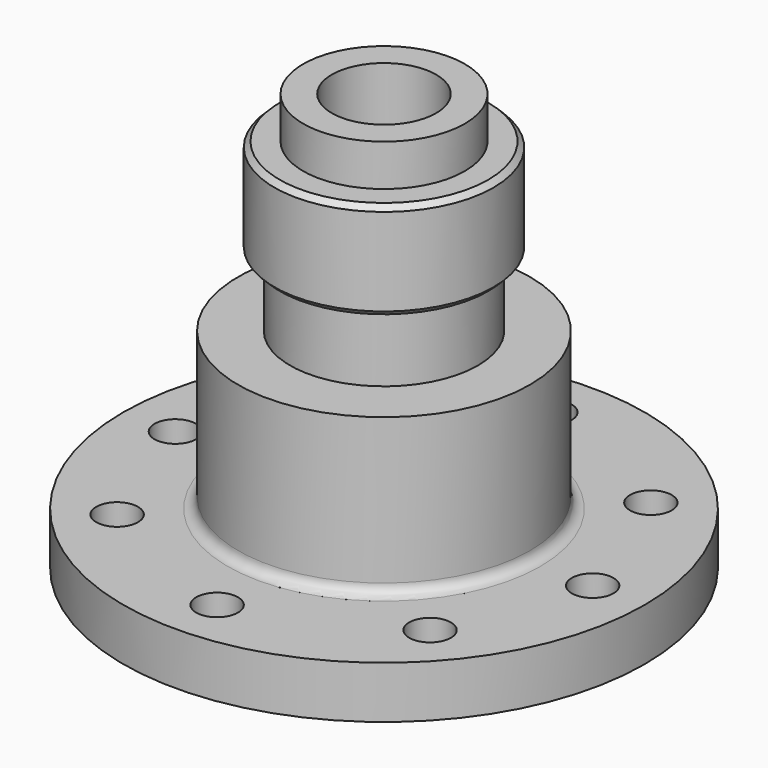
from build123d import *

# Parameters (mm, degrees)
F2_R     = 5
F3_DEPTH = 40
F2_R_2   = 11
F4_DEPTH = 9.6
F2_R_3   = 2
F5_DEPTH = 5
F6_SIZE  = 0.5
F7_SIZE2 = 0.5
F7_SIZE  = 0.5
F8_SIZE2 = 0.5
F8_SIZE  = 0.5


# Not quite as in the source:
# - a feature names something its author has since deleted; it is built from what else it names


with BuildPart() as f1:
    # F0 (on Front) → F1 (revolve)
    with BuildSketch(Plane.XZ):
        with BuildLine():
            Line((7.75, 0), (0, 0))
            Line((0, 0), (0, -40))
            Line((0, -40), (25, -40))
            Line((25, -40), (25, -35))
            Line((25, -35), (15, -35))
            ThreePointArc((15, -35), (14.2928932188, -34.7071067812), (14, -34))
            Line((14, -34), (14, -20))
            Line((14, -20), (9, -20))
            Line((9, -20), (9, -13.4))
            Line((9, -13.4), (10.5, -13.4))
            Line((10.5, -13.4), (10.5, -4))
            Line((10.5, -4), (7.75, -4))
            Line((7.75, -4), (7.75, 0))
        make_face()
    revolve(axis=Axis((0, 0, -20), (0, 0, 1)))

    # F2 (on face) → F3 (cut)
    with BuildSketch(Plane(origin=(0, 0, -40), x_dir=(1, 0, 0), z_dir=(0, 0, -1))):
        Circle(F2_R)
    extrude(amount=-F3_DEPTH, mode=Mode.SUBTRACT)

    # F2 (on face) → F4 (cut)
    with BuildSketch(Plane(origin=(0, 0, -40), x_dir=(1, 0, 0), z_dir=(0, 0, -1))):
        Circle(F2_R_2)
        Circle(F2_R, mode=Mode.SUBTRACT)
    extrude(amount=-F4_DEPTH, mode=Mode.SUBTRACT)

    # F2 (on face) → F5 (cut)
    with BuildSketch(Plane(origin=(0, 0, -40), x_dir=(1, 0, 0), z_dir=(0, 0, -1))):
        with Locations((15.0000959, 13.2286478141)):
            Circle(F2_R_3)
        with Locations((-15.0000959, 13.2286478141)):
            Circle(F2_R_3)
        with Locations((-15.0000959, -13.2286478141)):
            Circle(F2_R_3)
        with Locations((15.0000959, -13.2286478141)):
            Circle(F2_R_3)
        with Locations((0, -20)):
            Circle(F2_R_3)
        with Locations((20, 0)):
            Circle(F2_R_3)
        with Locations((-20, 0)):
            Circle(F2_R_3)
        with Locations((0, 20)):
            Circle(F2_R_3)
    extrude(amount=-F5_DEPTH, mode=Mode.SUBTRACT)

    # F6
    f6_edges = [f1.edges().sort_by_distance(p)[0] for p in [
        (-11, 0, -30.4),
    ]]
    chamfer(f6_edges, length=F6_SIZE)

    # F7
    f7_edges = [f1.edges().sort_by_distance(p)[0] for p in [
        (-10.5, 0, -13.4),
    ]]
    chamfer(f7_edges, length=F7_SIZE, length2=F7_SIZE2)

    # F8
    f8_edges = [f1.edges().sort_by_distance(p)[0] for p in [
        (-10.5, 0, -4),
    ]]
    chamfer(f8_edges, length=F8_SIZE, length2=F8_SIZE2)


solid = f1.part
